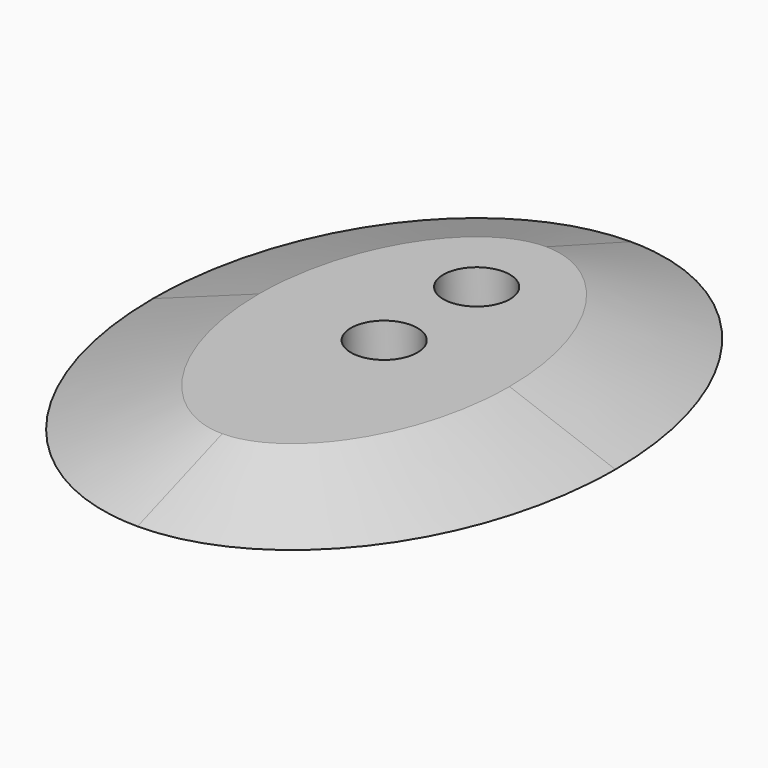
from build123d import *

# Parameters (mm, degrees)
F0_R     = 4.32
F1_DEPTH = 5
F1_TAPER = 70
F2_R     = 4.32
F3_DEPTH = 5


with BuildPart() as f1:
    # F0 (on Top) → F1 (new body)
    with BuildSketch(Plane.XY):
        with BuildLine():
            add(Edge.make_bspline(
                [(0, 40), (-51.961524, 40), (-25.980762, -20), (0, -80), (25.980762, -20), (51.961524, 40), (0, 40)],
                knots=[0, 0, 0, 2.094395, 2.094395, 4.18879, 4.18879, 6.283185, 6.283185, 6.283185], degree=2, weights=[1, 0.5, 1, 0.5, 1, 0.5, 1]))
        make_face()
        Circle(F0_R, mode=Mode.SUBTRACT)
        Circle(F0_R)
    extrude(amount=F1_DEPTH, taper=F1_TAPER)

    # F2 (on face) → F3 (cut, through all)
    with BuildSketch(Plane.XY.offset(5)):
        Circle(F2_R)
        with Locations((0, 15)):
            Circle(F2_R)
    extrude(amount=-F3_DEPTH, mode=Mode.SUBTRACT)


solid = f1.part
